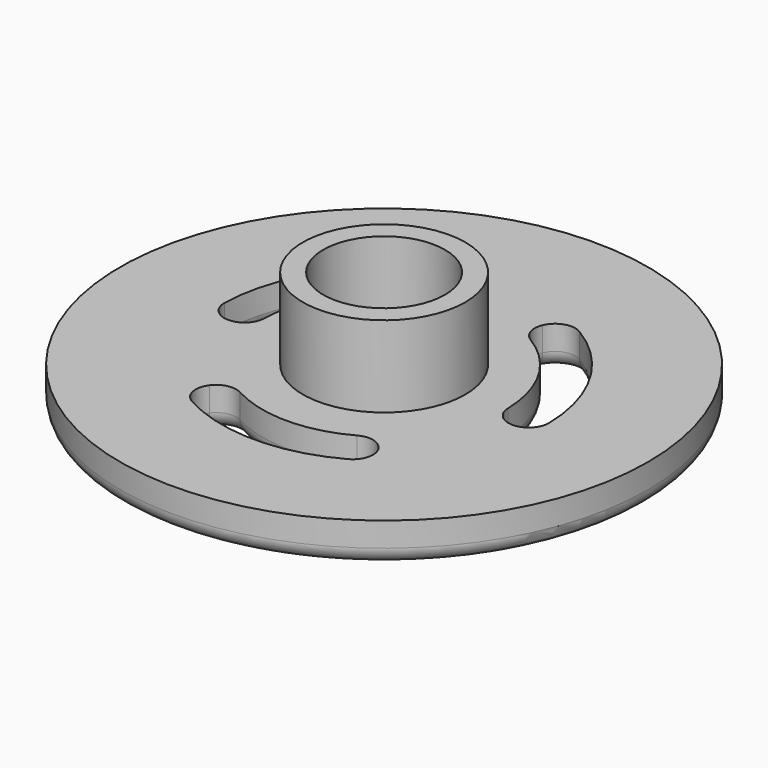
from build123d import *

# Parameters (mm, degrees)
F0_R     = 32.5
F1_DEPTH = 5
F2_R     = 10
F2_R_2   = 7.5
F3_DEPTH = 15
F4_R     = 2


with BuildPart() as f1:
    # F0 (on Top) → F1 (new body)
    with BuildSketch(Plane.XY):
        Circle(F0_R)
        with BuildLine():
            ThreePointArc((-9.6084106433, -17.5407652316), (-10.8510784968, -15.8756509046), (-10.4058874503, -13.8462090975))
            ThreePointArc((-10.4058874503, -13.8462090975), (-8.9348406398, -12.9044503937), (-7.2063079825, -13.1555739237))
            ThreePointArc((-7.2063079825, -13.1555739237), (0, -15), (7.2063079825, -13.1555739237))
            ThreePointArc((7.2063079825, -13.1555739237), (8.9348406398, -12.9044503937), (10.4058874503, -13.8462090975))
            ThreePointArc((10.4058874503, -13.8462090975), (10.8510784968, -15.8756509046), (9.6084106433, -17.5407652316))
            ThreePointArc((9.6084106433, -17.5407652316), (0, -20), (-9.6084106433, -17.5407652316))
        make_face(mode=Mode.SUBTRACT)
        with BuildLine():
            ThreePointArc((-19.994953614, 0.4492549087), (-17.3205080757, 10), (-10.3865429707, 17.0915103229))
            ThreePointArc((-10.3865429707, 17.0915103229), (-8.3231777366, 17.335135089), (-6.7882250994, 15.9348674296))
            ThreePointArc((-6.7882250994, 15.9348674296), (-6.708161543, 14.1900241697), (-7.789907228, 12.8186327422))
            ThreePointArc((-7.789907228, 12.8186327422), (-12.9903810568, 7.5), (-14.9962152105, 0.3369411815))
            ThreePointArc((-14.9962152105, 0.3369411815), (-15.6430021828, -1.285573776), (-17.1941125497, -2.0886583321))
            ThreePointArc((-17.1941125497, -2.0886583321), (-19.1742562334, -1.4594841844), (-19.994953614, 0.4492549087))
        make_face(mode=Mode.SUBTRACT)
        with BuildLine():
            ThreePointArc((0, 10), (7.0710678119, 7.0710678119), (10, 0))
            ThreePointArc((10, 0), (9.6592582629, -2.588190451), (8.6602540378, -5))
            ThreePointArc((8.6602540378, -5), (0, -10), (-8.6602540378, -5))
            ThreePointArc((-8.6602540378, -5), (-8.6602540378, 5), (0, 10))
        make_face(mode=Mode.SUBTRACT)
        with BuildLine():
            ThreePointArc((19.994953614, 0.4492549087), (19.1742562334, -1.4594841844), (17.1941125497, -2.0886583321))
            ThreePointArc((17.1941125497, -2.0886583321), (15.6430021828, -1.285573776), (14.9962152105, 0.3369411815))
            ThreePointArc((14.9962152105, 0.3369411815), (12.9903810568, 7.5), (7.789907228, 12.8186327422))
            ThreePointArc((7.789907228, 12.8186327422), (6.708161543, 14.1900241697), (6.7882250994, 15.9348674296))
            ThreePointArc((6.7882250994, 15.9348674296), (8.3231777366, 17.335135089), (10.3865429707, 17.0915103229))
            ThreePointArc((10.3865429707, 17.0915103229), (17.3205080757, 10), (19.994953614, 0.4492549087))
        make_face(mode=Mode.SUBTRACT)
    extrude(amount=F1_DEPTH)

    # F2 (on face) → F3 (join)
    with BuildSketch(Plane(origin=(0, 0, 0), x_dir=(1, 0, 0), z_dir=(0, 0, -1))):
        Circle(F2_R)
        Circle(F2_R_2, mode=Mode.SUBTRACT)
    extrude(amount=-F3_DEPTH)

    # F4
    f4_edges = [f1.edges().sort_by_distance(p)[0] for p in [
        (-32.5, 0, 0),
        (-10.599955, -14.147118, 0),
        (0, -15, 0),
        (10.599955, -14.147118, 0),
        (0, -20, 0),
        (-17.551741, -2.106271, 0),
        (-17.320508, 10, 0),
        (-6.951786, 16.253389, 0),
        (-12.990381, 7.5, 0),
        (17.320508, 10, 0),
        (17.551741, -2.106271, 0),
        (12.990381, 7.5, 0),
        (6.951786, 16.253389, 0),
        (-7.5, 0, 0),
    ]]
    fillet(f4_edges, radius=F4_R)


solid = f1.part
